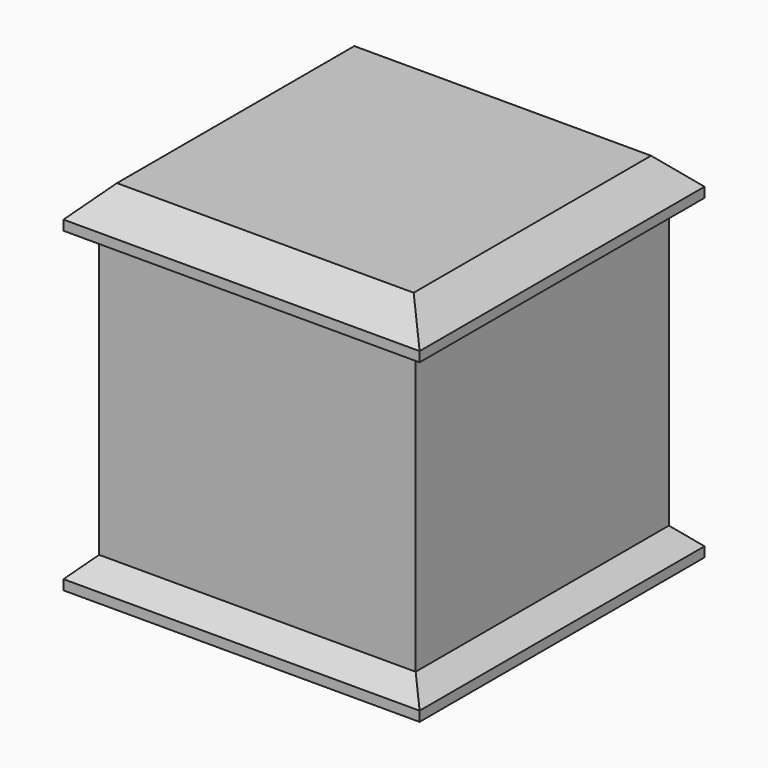
from build123d import *

# Parameters (mm, degrees)
F0_W          = 101.6
F0_H          = 6.35
F0_H_2        = 88.9
F1_DEPTH      = 50.8
F2_DEPTH      = 57.15
F3_DEPTH      = 57.15
F4_T1_DEPTH   = 163.2905609208
F4_T3_DEPTH   = 163.2905609208
F4_T8_DEPTH   = 163.2905609208
F4_T14_DEPTH  = 163.2905609208
F4_T20_DEPTH  = 163.2905609208
F4_T27_DEPTH  = 163.2905609208
F4_T33_DEPTH  = 163.2905609208
F4_T39_DEPTH  = 163.2905609208
F4_T45_DEPTH  = 163.2905609208
F4_T51_DEPTH  = 163.2905609208
F4_T58_DEPTH  = 163.2905609208
F4_T64_DEPTH  = 163.2905609208
F4_T70_DEPTH  = 163.2905609208
F4_T76_DEPTH  = 163.2905609208
F4_T82_DEPTH  = 163.2905609208
F4_T89_DEPTH  = 163.2905609208
F4_T95_DEPTH  = 163.2905609208
F4_T101_DEPTH = 163.2905609208
F4_T107_DEPTH = 163.2905609208
F4_T113_DEPTH = 163.2905609208
F4_T120_DEPTH = 163.2905609208
F4_T126_DEPTH = 163.2905609208


# Not quite as in the source:
# - a fillet or chamfer that OpenCascade refuses, or shapes differently, is made with other operations: its cross-section is extruded or revolved along the edge and cut away or added


with BuildPart() as f1:
    # F0 (on Front) → F1 (new body, symmetric)
    with BuildSketch(Plane.XZ):
        with Locations((0, -47.625)):
            Rectangle(F0_W, F0_H)
        Rectangle(F0_W, F0_H_2)
        with Locations((0, 47.625)):
            Rectangle(F0_W, F0_H)
    extrude(amount=F1_DEPTH, both=True)

    # F0 (on Front) → F2 (join, symmetric)
    with BuildSketch(Plane.XZ):
        Polygon((-50.8, 44.45), (-50.8, 50.8), (50.8, 50.8), (50.8, 44.45), (57.15, 44.45), (57.15, 57.15), (-57.15, 57.15), (-57.15, 44.45), align=None)
        Polygon((-50.8, -50.8), (-50.8, -44.45), (-57.15, -44.45), (-57.15, -57.15), (57.15, -57.15), (57.15, -44.45), (50.8, -44.45), (50.8, -50.8), align=None)
    extrude(amount=F2_DEPTH, both=True)

    # F0 (on Front) → F3 (join, symmetric)
    with BuildSketch(Plane.XZ):
        with Locations((0, 47.625)):
            Rectangle(F0_W, F0_H)
        with Locations((0, -47.625)):
            Rectangle(F0_W, F0_H)
    extrude(amount=F3_DEPTH, both=True)

    # F4: chamfer of 9.525 on 8 edges, made by hand

    # F4_s2 → F4_t1 (cut)
    with BuildSketch(Plane.YZ.offset(-81.6452804604)):
        Polygon((-47.625, 57.15), (-57.15, 47.625), (-57.15, 57.15), align=None)
        Polygon((47.625, 57.15), (57.15, 47.625), (57.15, 57.15), align=None)
    extrude(amount=F4_T1_DEPTH, mode=Mode.SUBTRACT)

    # F4_s4 → F4_t3 (cut)
    with BuildSketch(Plane.XZ.offset(-81.6452804604)):
        Polygon((47.625, 57.15), (57.15, 47.625), (57.15, 57.15), align=None)
        Polygon((-57.15, 47.625), (-47.625, 57.15), (-57.15, 57.15), align=None)
    extrude(amount=F4_T3_DEPTH, mode=Mode.SUBTRACT)


with BuildPart() as f4_tool6:
    # F4_s7 → F4_t8 (new body)
    with BuildSketch(Plane.XZ.offset(81.6452804604)):
        Polygon((47.625, -44.45), (57.15, -53.975), (57.15, -44.45), align=None)
    extrude(amount=-F4_T8_DEPTH)

    split(bisect_by=Plane.YZ.offset(50.8), keep=Keep.BOTTOM)

    split(bisect_by=Plane.XZ.offset(50.8), keep=Keep.TOP)


with BuildPart() as f1_1:
    add(f1.part)

    # F4_t5: cut F4_tool6
    add(f4_tool6.part, mode=Mode.SUBTRACT)


with BuildPart() as f4_tool12:
    # F4_s13 → F4_t14 (new body)
    with BuildSketch(Plane.XZ.offset(81.6452804604)):
        Polygon((47.625, -44.45), (57.15, -53.975), (57.15, -44.45), align=None)
    extrude(amount=-F4_T14_DEPTH)

    split(bisect_by=Plane.YZ.offset(50.8), keep=Keep.TOP)

    split(bisect_by=Plane.XZ.offset(50.8), keep=Keep.TOP)


with BuildPart() as f1_2:
    add(f1_1.part)

    # F4_t11: cut F4_tool12
    add(f4_tool12.part, mode=Mode.SUBTRACT)


with BuildPart() as f4_tool18:
    # F4_s19 → F4_t20 (new body)
    with BuildSketch(Plane.XZ.offset(81.6452804604)):
        Polygon((47.625, -44.45), (57.15, -53.975), (57.15, -44.45), align=None)
    extrude(amount=-F4_T20_DEPTH)

    split(bisect_by=Plane.XZ.offset(-50.8), keep=Keep.TOP)

    split(bisect_by=Plane.YZ.offset(50.8), keep=Keep.TOP)

    split(bisect_by=Plane.XZ.offset(50.8), keep=Keep.BOTTOM)


with BuildPart() as f1_3:
    add(f1_2.part)

    # F4_t17: cut F4_tool18
    add(f4_tool18.part, mode=Mode.SUBTRACT)


with BuildPart() as f4_tool25:
    # F4_s26 → F4_t27 (new body)
    with BuildSketch(Plane.XZ.offset(81.6452804604)):
        Polygon((47.625, -44.45), (57.15, -53.975), (57.15, -44.45), align=None)
    extrude(amount=-F4_T27_DEPTH)

    split(bisect_by=Plane.XZ.offset(-50.8), keep=Keep.BOTTOM)

    split(bisect_by=Plane.YZ.offset(50.8), keep=Keep.BOTTOM)


with BuildPart() as f1_4:
    add(f1_3.part)

    # F4_t24: cut F4_tool25
    add(f4_tool25.part, mode=Mode.SUBTRACT)


with BuildPart() as f4_tool31:
    # F4_s32 → F4_t33 (new body)
    with BuildSketch(Plane.XZ.offset(81.6452804604)):
        Polygon((47.625, -44.45), (57.15, -53.975), (57.15, -44.45), align=None)
    extrude(amount=-F4_T33_DEPTH)

    split(bisect_by=Plane.XZ.offset(-50.8), keep=Keep.BOTTOM)

    split(bisect_by=Plane.YZ.offset(50.8), keep=Keep.TOP)


with BuildPart() as f1_5:
    add(f1_4.part)

    # F4_t30: cut F4_tool31
    add(f4_tool31.part, mode=Mode.SUBTRACT)


with BuildPart() as f4_tool37:
    # F4_s38 → F4_t39 (new body)
    with BuildSketch(Plane.YZ.offset(-81.6452804604)):
        Polygon((-47.625, -44.45), (-57.15, -53.975), (-57.15, -44.45), align=None)
    extrude(amount=F4_T39_DEPTH)

    split(bisect_by=Plane.YZ.offset(-50.8), keep=Keep.BOTTOM)

    split(bisect_by=Plane.XZ.offset(50.8), keep=Keep.BOTTOM)


with BuildPart() as f1_6:
    add(f1_5.part)

    # F4_t36: cut F4_tool37
    add(f4_tool37.part, mode=Mode.SUBTRACT)


with BuildPart() as f4_tool43:
    # F4_s44 → F4_t45 (new body)
    with BuildSketch(Plane.YZ.offset(-81.6452804604)):
        Polygon((-47.625, -44.45), (-57.15, -53.975), (-57.15, -44.45), align=None)
    extrude(amount=F4_T45_DEPTH)

    split(bisect_by=Plane.YZ.offset(-50.8), keep=Keep.BOTTOM)

    split(bisect_by=Plane.XZ.offset(50.8), keep=Keep.TOP)


with BuildPart() as f1_7:
    add(f1_6.part)

    # F4_t42: cut F4_tool43
    add(f4_tool43.part, mode=Mode.SUBTRACT)


with BuildPart() as f4_tool49:
    # F4_s50 → F4_t51 (new body)
    with BuildSketch(Plane.YZ.offset(-81.6452804604)):
        Polygon((-47.625, -44.45), (-57.15, -53.975), (-57.15, -44.45), align=None)
    extrude(amount=F4_T51_DEPTH)

    split(bisect_by=Plane.YZ.offset(-50.8), keep=Keep.TOP)

    split(bisect_by=Plane.YZ.offset(50.8), keep=Keep.BOTTOM)

    split(bisect_by=Plane.XZ.offset(50.8), keep=Keep.TOP)


with BuildPart() as f1_8:
    add(f1_7.part)

    # F4_t48: cut F4_tool49
    add(f4_tool49.part, mode=Mode.SUBTRACT)


with BuildPart() as f4_tool56:
    # F4_s57 → F4_t58 (new body)
    with BuildSketch(Plane.YZ.offset(-81.6452804604)):
        Polygon((-47.625, -44.45), (-57.15, -53.975), (-57.15, -44.45), align=None)
    extrude(amount=F4_T58_DEPTH)

    split(bisect_by=Plane.YZ.offset(50.8), keep=Keep.TOP)

    split(bisect_by=Plane.XZ.offset(50.8), keep=Keep.BOTTOM)


with BuildPart() as f1_9:
    add(f1_8.part)

    # F4_t55: cut F4_tool56
    add(f4_tool56.part, mode=Mode.SUBTRACT)


with BuildPart() as f4_tool62:
    # F4_s63 → F4_t64 (new body)
    with BuildSketch(Plane.YZ.offset(-81.6452804604)):
        Polygon((-47.625, -44.45), (-57.15, -53.975), (-57.15, -44.45), align=None)
    extrude(amount=F4_T64_DEPTH)

    split(bisect_by=Plane.YZ.offset(50.8), keep=Keep.TOP)

    split(bisect_by=Plane.XZ.offset(50.8), keep=Keep.TOP)


with BuildPart() as f1_10:
    add(f1_9.part)

    # F4_t61: cut F4_tool62
    add(f4_tool62.part, mode=Mode.SUBTRACT)


with BuildPart() as f4_tool68:
    # F4_s69 → F4_t70 (new body)
    with BuildSketch(Plane.XZ.offset(-81.6452804604)):
        Polygon((-47.625, -44.45), (-57.15, -53.975), (-57.15, -44.45), align=None)
    extrude(amount=F4_T70_DEPTH)

    split(bisect_by=Plane.YZ.offset(-50.8), keep=Keep.TOP)

    split(bisect_by=Plane.XZ.offset(-50.8), keep=Keep.BOTTOM)


with BuildPart() as f1_11:
    add(f1_10.part)

    # F4_t67: cut F4_tool68
    add(f4_tool68.part, mode=Mode.SUBTRACT)


with BuildPart() as f4_tool74:
    # F4_s75 → F4_t76 (new body)
    with BuildSketch(Plane.XZ.offset(-81.6452804604)):
        Polygon((-47.625, -44.45), (-57.15, -53.975), (-57.15, -44.45), align=None)
    extrude(amount=F4_T76_DEPTH)

    split(bisect_by=Plane.YZ.offset(-50.8), keep=Keep.BOTTOM)

    split(bisect_by=Plane.XZ.offset(-50.8), keep=Keep.BOTTOM)


with BuildPart() as f1_12:
    add(f1_11.part)

    # F4_t73: cut F4_tool74
    add(f4_tool74.part, mode=Mode.SUBTRACT)


with BuildPart() as f4_tool80:
    # F4_s81 → F4_t82 (new body)
    with BuildSketch(Plane.XZ.offset(-81.6452804604)):
        Polygon((-47.625, -44.45), (-57.15, -53.975), (-57.15, -44.45), align=None)
    extrude(amount=F4_T82_DEPTH)

    split(bisect_by=Plane.YZ.offset(-50.8), keep=Keep.BOTTOM)

    split(bisect_by=Plane.XZ.offset(-50.8), keep=Keep.TOP)

    split(bisect_by=Plane.XZ.offset(50.8), keep=Keep.BOTTOM)


with BuildPart() as f1_13:
    add(f1_12.part)

    # F4_t79: cut F4_tool80
    add(f4_tool80.part, mode=Mode.SUBTRACT)


with BuildPart() as f4_tool87:
    # F4_s88 → F4_t89 (new body)
    with BuildSketch(Plane.XZ.offset(-81.6452804604)):
        Polygon((-47.625, -44.45), (-57.15, -53.975), (-57.15, -44.45), align=None)
    extrude(amount=F4_T89_DEPTH)

    split(bisect_by=Plane.YZ.offset(-50.8), keep=Keep.TOP)

    split(bisect_by=Plane.XZ.offset(50.8), keep=Keep.TOP)


with BuildPart() as f1_14:
    add(f1_13.part)

    # F4_t86: cut F4_tool87
    add(f4_tool87.part, mode=Mode.SUBTRACT)


with BuildPart() as f4_tool93:
    # F4_s94 → F4_t95 (new body)
    with BuildSketch(Plane.XZ.offset(-81.6452804604)):
        Polygon((-47.625, -44.45), (-57.15, -53.975), (-57.15, -44.45), align=None)
    extrude(amount=F4_T95_DEPTH)

    split(bisect_by=Plane.YZ.offset(-50.8), keep=Keep.BOTTOM)

    split(bisect_by=Plane.XZ.offset(50.8), keep=Keep.TOP)


with BuildPart() as f1_15:
    add(f1_14.part)

    # F4_t92: cut F4_tool93
    add(f4_tool93.part, mode=Mode.SUBTRACT)


with BuildPart() as f4_tool99:
    # F4_s100 → F4_t101 (new body)
    with BuildSketch(Plane.YZ.offset(81.6452804604)):
        Polygon((47.625, -44.45), (57.15, -53.975), (57.15, -44.45), align=None)
    extrude(amount=-F4_T101_DEPTH)

    split(bisect_by=Plane.XZ.offset(-50.8), keep=Keep.TOP)

    split(bisect_by=Plane.YZ.offset(50.8), keep=Keep.TOP)


with BuildPart() as f1_16:
    add(f1_15.part)

    # F4_t98: cut F4_tool99
    add(f4_tool99.part, mode=Mode.SUBTRACT)


with BuildPart() as f4_tool105:
    # F4_s106 → F4_t107 (new body)
    with BuildSketch(Plane.YZ.offset(81.6452804604)):
        Polygon((47.625, -44.45), (57.15, -53.975), (57.15, -44.45), align=None)
    extrude(amount=-F4_T107_DEPTH)

    split(bisect_by=Plane.XZ.offset(-50.8), keep=Keep.BOTTOM)

    split(bisect_by=Plane.YZ.offset(50.8), keep=Keep.TOP)


with BuildPart() as f1_17:
    add(f1_16.part)

    # F4_t104: cut F4_tool105
    add(f4_tool105.part, mode=Mode.SUBTRACT)


with BuildPart() as f4_tool111:
    # F4_s112 → F4_t113 (new body)
    with BuildSketch(Plane.YZ.offset(81.6452804604)):
        Polygon((47.625, -44.45), (57.15, -53.975), (57.15, -44.45), align=None)
    extrude(amount=-F4_T113_DEPTH)

    split(bisect_by=Plane.YZ.offset(-50.8), keep=Keep.TOP)

    split(bisect_by=Plane.XZ.offset(-50.8), keep=Keep.BOTTOM)

    split(bisect_by=Plane.YZ.offset(50.8), keep=Keep.BOTTOM)


with BuildPart() as f1_18:
    add(f1_17.part)

    # F4_t110: cut F4_tool111
    add(f4_tool111.part, mode=Mode.SUBTRACT)


with BuildPart() as f4_tool118:
    # F4_s119 → F4_t120 (new body)
    with BuildSketch(Plane.YZ.offset(81.6452804604)):
        Polygon((47.625, -44.45), (57.15, -53.975), (57.15, -44.45), align=None)
    extrude(amount=-F4_T120_DEPTH)

    split(bisect_by=Plane.YZ.offset(-50.8), keep=Keep.BOTTOM)

    split(bisect_by=Plane.XZ.offset(-50.8), keep=Keep.TOP)


with BuildPart() as f1_19:
    add(f1_18.part)

    # F4_t117: cut F4_tool118
    add(f4_tool118.part, mode=Mode.SUBTRACT)


with BuildPart() as f4_tool124:
    # F4_s125 → F4_t126 (new body)
    with BuildSketch(Plane.YZ.offset(81.6452804604)):
        Polygon((47.625, -44.45), (57.15, -53.975), (57.15, -44.45), align=None)
    extrude(amount=-F4_T126_DEPTH)

    split(bisect_by=Plane.YZ.offset(-50.8), keep=Keep.BOTTOM)

    split(bisect_by=Plane.XZ.offset(-50.8), keep=Keep.BOTTOM)


with BuildPart() as f1_20:
    add(f1_19.part)

    # F4_t123: cut F4_tool124
    add(f4_tool124.part, mode=Mode.SUBTRACT)


solid = f1_20.part
